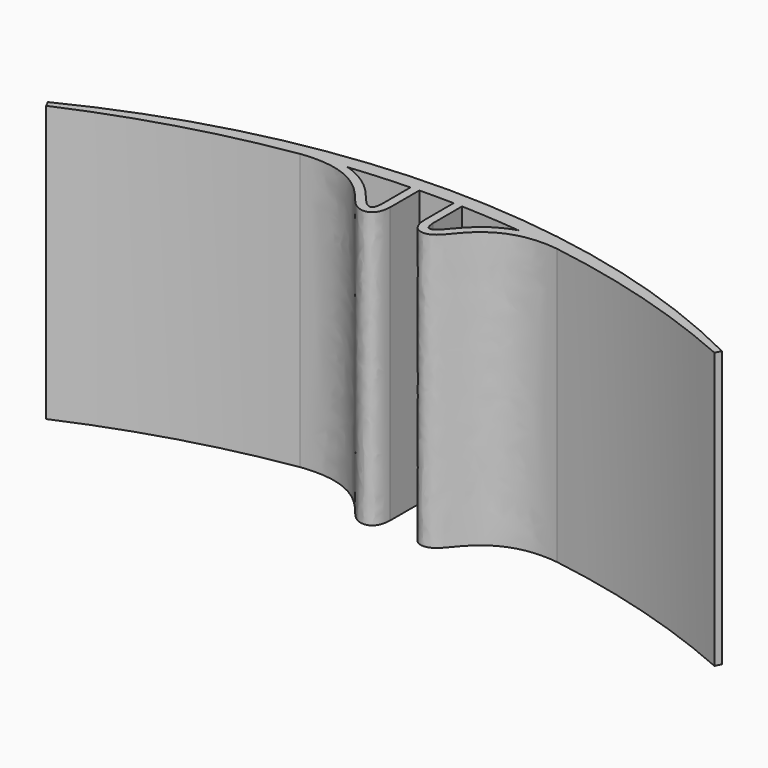
from build123d import *

# Parameters (mm, degrees)
F1_DEPTH = 45


# Not quite as in the source:
# - ends of sketch curves that miss each other by under 0.0002 mm in the source are joined
# - the dataset's text gives a spline's control points without its knots; the knots are read off the source's solid


with BuildPart() as f1:
    # F0 (on Top) → F1 (new body)
    with BuildSketch(Plane.XY):
        with BuildLine():
            add(Edge.make_bspline(
                [(2.8, 4.55), (2.9339124449, 1.7287548399), (6.1294716036, 1.1822923466), (8.6407401327, 5.2198615541), (13.9829784257, 9.8247092009), (20.9692498837, 8.9133747947)],
                knots=[0, 0, 0, 0, 0.2609361061, 0.5223940983, 1, 1, 1, 1], degree=3))
            ThreePointArc((20.9692498837, 8.9133747947), (17.453741319, 9.4182639689), (13.9261800828, 9.8306051768))
            add(Edge.make_bspline(
                [(4.20000081, 4.5849169776), (4.2137809328, 4.3234076056), (4.2725955516, 3.8743004851), (4.4118012954, 3.4443453717), (4.5451673752, 3.2307676133), (4.6271725043, 3.1584792767), (4.6823628614, 3.1287706535), (4.7756356234, 3.1041431218), (4.9314555103, 3.1024294358), (5.0957052816, 3.1340941468), (5.2288051779, 3.1779244701), (5.3546254511, 3.2305198956), (5.5102903775, 3.3165940703), (5.7159083264, 3.4683572028), (6.0258328333, 3.7515004168), (6.4831199341, 4.267856579), (7.1599996258, 5.106923618), (8.0189640554, 6.0946683852), (9.0819782359, 7.1365991751), (10.3791905584, 8.160200297), (11.9634714653, 9.1034905452), (13.2258849115, 9.614435556), (13.9261800828, 9.8306051768)],
                knots=[0.0011975807, 0.0011975807, 0.0011975807, 0.0011975807, 0.03125, 0.0625, 0.09375, 0.125, 0.15625, 0.1875, 0.21875, 0.25, 0.265625, 0.28125, 0.3125, 0.34375, 0.375, 0.4375, 0.5, 0.5625, 0.625, 0.6875, 0.75, 0.8156240768, 0.8156240768, 0.8156240768, 0.8156240768], degree=3))
            Line((4.20000081, 4.5849169776), (4.2, 10.4847246236))
            ThreePointArc((4.2, 10.4847246236), (3.5000469771, 10.5046720065), (2.8, 10.5209926146))
            Line((2.8, 10.5209926146), (2.8, 4.55))
        make_face()
        with BuildLine():
            ThreePointArc((-13.9261800828, 9.8306051768), (-17.453741319, 9.4182639689), (-20.9692498837, 8.9133747947))
            add(Edge.make_bspline(
                [(-2.8, 4.55), (-2.9339124449, 1.7287548399), (-6.1294716036, 1.1822923466), (-8.6407401327, 5.2198615541), (-13.9829784257, 9.8247092009), (-20.9692498837, 8.9133747947)],
                knots=[0, 0, 0, 0, 0.2609361061, 0.5223940983, 1, 1, 1, 1], degree=3))
            Line((-2.8, 4.55), (-2.8, 10.5209926146))
            ThreePointArc((-2.8, 10.5209926146), (-3.5000469771, 10.5046720065), (-4.2, 10.4847246236))
            Line((-4.2, 10.4847246236), (-4.2, 4.5849169349))
            add(Edge.make_bspline(
                [(-4.2, 4.5849169349), (-4.2137809328, 4.3234076056), (-4.2725955516, 3.8743004851), (-4.4118012954, 3.4443453717), (-4.5451673752, 3.2307676133), (-4.6271725043, 3.1584792767), (-4.6823628614, 3.1287706535), (-4.7756356234, 3.1041431218), (-4.9314555103, 3.1024294358), (-5.0957052816, 3.1340941468), (-5.2288051779, 3.1779244701), (-5.3546254511, 3.2305198956), (-5.5102903774, 3.3165940703), (-5.7159083264, 3.4683572028), (-6.0258328333, 3.7515004168), (-6.4831199341, 4.267856579), (-7.1599996258, 5.106923618), (-8.0189640554, 6.0946683852), (-9.0819782359, 7.1365991751), (-10.3791905583, 8.160200297), (-11.9634714653, 9.1034905452), (-13.2258849115, 9.614435556), (-13.9261800828, 9.8306051768)],
                knots=[0.0011975807, 0.0011975807, 0.0011975807, 0.0011975807, 0.03125, 0.0625, 0.09375, 0.125, 0.15625, 0.1875, 0.21875, 0.25, 0.265625, 0.28125, 0.3125, 0.34375, 0.375, 0.4375, 0.5, 0.5625, 0.625, 0.6875, 0.75, 0.8156240768, 0.8156240768, 0.8156240768, 0.8156240768], degree=3))
        make_face()
        with BuildLine():
            Line((54.5299840881, -0.9389276024), (55, 0))
            ThreePointArc((55, 0), (0, 13), (-55, 0))
            Line((-55, 0), (-54.5299840881, -0.9389276024))
            ThreePointArc((-54.5299840881, -0.9389276024), (-38.0696801696, 5.0774819949), (-20.9692498837, 8.9133747947))
            ThreePointArc((-20.9692498837, 8.9133747947), (-17.453741319, 9.4182639689), (-13.9261800828, 9.8306051768))
            ThreePointArc((-13.9261800828, 9.8306051768), (-9.0689894234, 10.2453835144), (-4.2, 10.4847246236))
            ThreePointArc((-4.2, 10.4847246236), (-3.5000469771, 10.5046720065), (-2.8, 10.5209926146))
            ThreePointArc((-2.8, 10.5209926146), (0, 10.55), (2.8, 10.5209926146))
            ThreePointArc((2.8, 10.5209926146), (3.5000469771, 10.5046720065), (4.2, 10.4847246236))
            ThreePointArc((4.2, 10.4847246236), (9.0689894234, 10.2453835144), (13.9261800828, 9.8306051768))
            ThreePointArc((13.9261800828, 9.8306051768), (17.453741319, 9.4182639689), (20.9692498837, 8.9133747947))
            ThreePointArc((20.9692498837, 8.9133747947), (38.0696801696, 5.0774819949), (54.5299840881, -0.9389276024))
        make_face()
    extrude(amount=F1_DEPTH)


solid = f1.part
